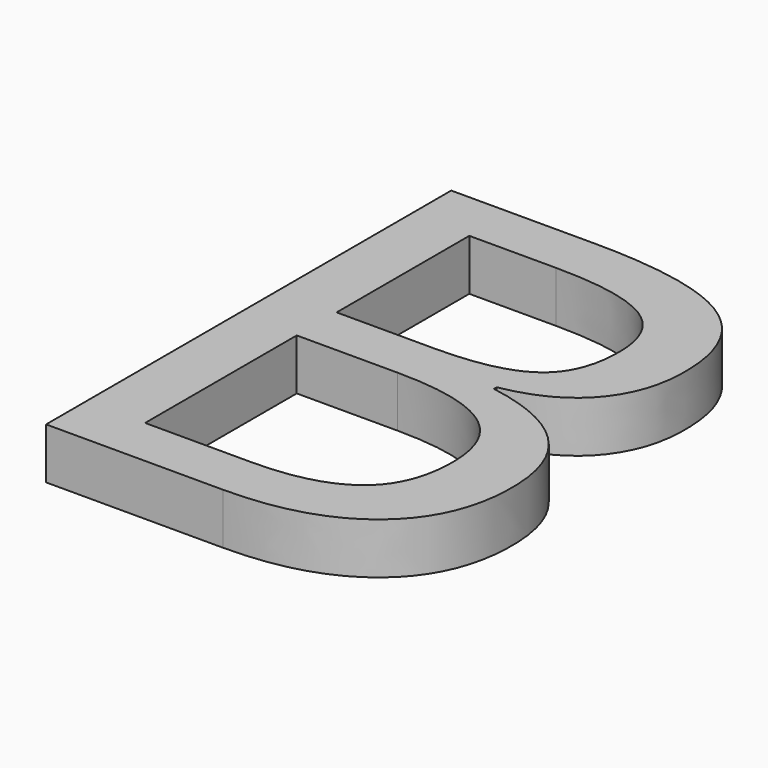
from build123d import *

# Parameters (mm, degrees)
F0_TEXT_SIZE = 41.6666666667
F1_DEPTH     = 3


# Not quite as in the source:
# - Text() gives the source's letters only with a copy of the font that has no kerning and outlines rounded to 1/6400 em; it was checked with that copy


with BuildPart() as f1:
    # F0 (on Top) → F1 (new body)
    with BuildSketch(Plane.XY):
        with Locations((0, 0)):
            Text('B', F0_TEXT_SIZE, font='Open Sans', text_align=(TextAlign.LEFT, TextAlign.BOTTOM))
    extrude(amount=F1_DEPTH)


solid = f1.part
